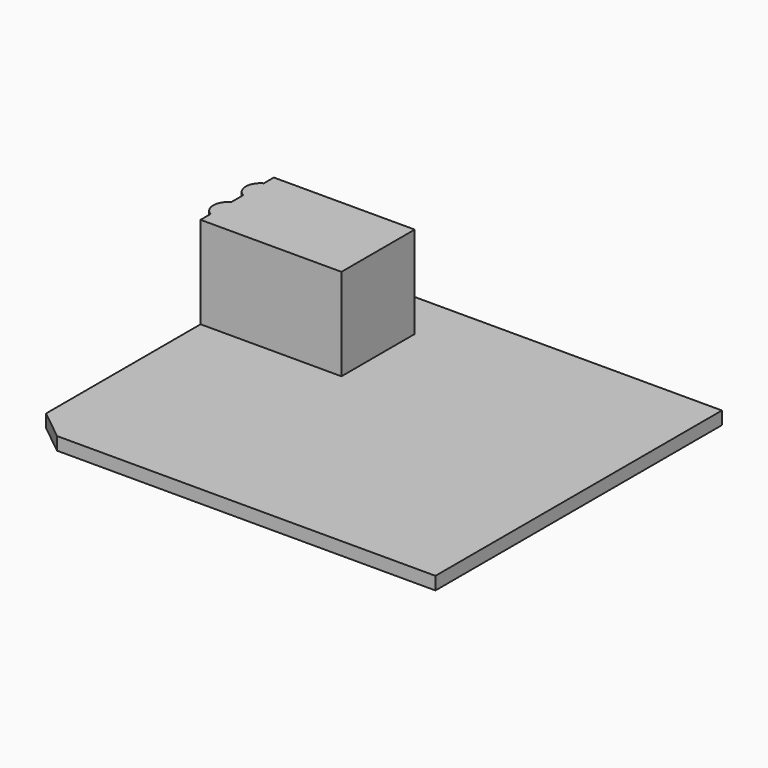
from build123d import *

# Parameters (mm, degrees)
F1_DEPTH = 1.6764
F3_DEPTH = 11.938
F4_W     = 10.033
F4_H     = 5.08
F5_DEPTH = 6.5278


with BuildPart() as f1:
    # F0 (on Top) → F1 (new body)
    with BuildSketch(Plane.XY):
        Polygon((-22.5799904745, -23.241), (26.543, -23.241), (26.543, 23.241), (-22.5799904745, 23.241), (-26.543, 20.062799959), (-26.543, -20.062799959), align=None)
    extrude(amount=F1_DEPTH)

    # F2 (on face) → F3 (join)
    with BuildSketch(Plane.XY.offset(1.6764)):
        with BuildLine():
            Line((-26.543, 6.6294), (-26.543, 5.0038))
            Line((-26.543, 5.0038), (-8.255, 5.0038))
            Line((-8.255, 5.0038), (-8.255, 16.891))
            Line((-8.255, 16.891), (-26.543, 16.891))
            Line((-26.543, 16.891), (-26.543, 15.2654))
            ThreePointArc((-26.543, 15.2654), (-27.5392260553, 13.5911375004), (-26.543, 11.9168750008))
            Line((-26.543, 11.9168750008), (-26.543, 9.967618097))
            ThreePointArc((-26.543, 9.967618097), (-27.5297952384, 8.2985090485), (-26.543, 6.6294))
        make_face()
    extrude(amount=F3_DEPTH)

    # F4 (on face) → F5 (join)
    with BuildSketch(Plane(origin=(0, 0, 0), x_dir=(1, 0, 0), z_dir=(0, 0, -1))):
        with Locations((-19.9928638897, -13.5961750215)):
            Rectangle(F4_W, F4_H)
        with Locations((-19.9928638897, -6.4841750215)):
            Rectangle(F4_W, F4_H)
    extrude(amount=F5_DEPTH)


solid = f1.part
